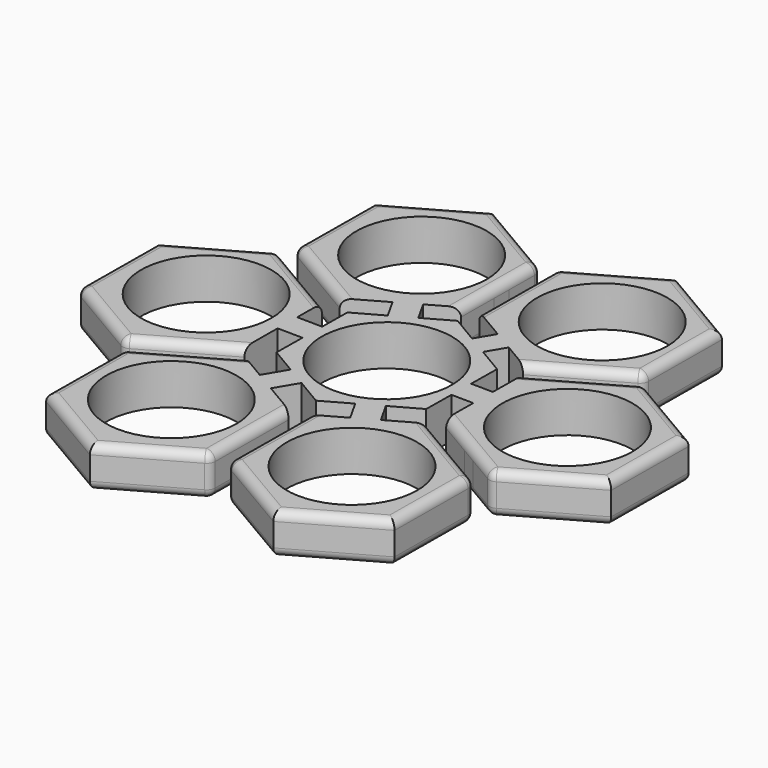
from build123d import *

# Parameters (mm, degrees)
F0_R          = 11.2
F1_DEPTH      = 7
F2_R          = 1.5
F3_R          = 1.5
F4_T1_DEPTH   = 19.3547728944
F4_T3_DEPTH   = 19.3547728944
F4_T5_DEPTH   = 19.3547728944
F4_T7_DEPTH   = 19.3547728944
F4_T9_DEPTH   = 19.3547728944
F4_T11_DEPTH  = 19.3547728944
F4_T13_DEPTH  = 19.3547728944
F4_T15_DEPTH  = 19.3547728944
F4_T17_DEPTH  = 19.3547728944
F4_T19_DEPTH  = 19.3547728944
F4_T21_DEPTH  = 19.3547728944
F4_T23_DEPTH  = 19.3547728944
F4_T25_DEPTH  = 4
F4_T27_DEPTH  = 7.6650635095
F4_T32_DEPTH  = 1.5
F4_T38_DEPTH  = 1.5
F4_T44_DEPTH  = 1.5
F4_T50_DEPTH  = 1.5
F4_T56_DEPTH  = 1.5
F4_T62_DEPTH  = 1.5
F4_T68_DEPTH  = 1.5
F4_T74_DEPTH  = 1.5
F4_T80_DEPTH  = 1.5
F4_T86_DEPTH  = 1.5
F4_T92_DEPTH  = 1.5
F4_T98_DEPTH  = 1.5
F4_T104_DEPTH = 1.5
F4_T110_DEPTH = 1.5
F4_T116_DEPTH = 1.5
F4_T122_DEPTH = 1.5
F4_T128_DEPTH = 1.5
F4_T134_DEPTH = 1.5
F4_T140_DEPTH = 1.5
F4_T146_DEPTH = 1.5
F4_T152_DEPTH = 1.5
F4_T158_DEPTH = 1.5
F4_T164_DEPTH = 1.5
F5_T1_DEPTH   = 14.7387474906
F5_T3_DEPTH   = 19.3547728944
F5_T5_DEPTH   = 4
F5_T10_DEPTH  = 1.5
F5_T16_DEPTH  = 1.5
F5_T20_ANGLE  = 60.0000000024


# Not quite as in the source:
# - a fillet or chamfer that OpenCascade refuses, or shapes differently, is made with other operations: its cross-section is extruded or revolved along the edge and cut away or added


with BuildPart() as f1:
    # F0 (on Top) → F1 (new body)
    with BuildSketch(Plane.XY):
        Polygon((-17.3645722709, -8.8701178063), (-17.3063848903, -1.7982007172), (-17.272166827, 2.3605585075), (-17.2290559521, 7.6001229905), (-25.7244198376, 12.5985677043), (-31.4249447291, 15.9526039637), (-45.7563498251, 7.8348441401), (-45.891866144, -8.6353966568), (-31.6959773669, -16.98787763), align=None)
        with Locations((-31.0137589486, 0)):
            Circle(F0_R, mode=Mode.SUBTRACT)
        Polygon((8.1018030655, -10.3313899594), (12.8824554247, -7.6483706617), (12.9474991031, -2.30788682), (12.9981476939, 1.8506722915), (13.064911003, 7.3323483301), (8.4724381667, 10.0589197287), (4.8963446285, 12.1820622508), (0.1824555782, 14.9807189918), (-4.4750609364, 12.3668065487), (-8.1018030655, 10.3313899594), (-12.8824554247, 7.6483706617), (-12.9474991031, 2.30788682), (-12.9981476939, -1.8506722915), (-13.064911003, -7.3323483301), (-8.4724381667, -10.0589197287), (-4.8963446285, -12.1820622508), (-0.1824555782, -14.9807189918), (4.4750609364, -12.3668065487), align=None)
        Circle(F0_R, mode=Mode.SUBTRACT)
        Polygon((-10.0334618511, 13.7732545552), (-6.4147616826, 15.8230004555), (-1.9451605955, 18.3547234715), (-1.8875629406, 25.354967087), (-1.8610559953, 28.5765405116), (-1.8096442766, 34.8249642683), (-16.0055330537, 43.1774452415), (-30.3369381496, 35.0596854179), (-30.4724544685, 18.589444621), (-16.2765656915, 10.2369636478), align=None)
        with Locations((-15.5068794743, 26.8587031163)):
            Circle(F0_R, mode=Mode.SUBTRACT)
        Polygon((6.7727997891, 15.3426504379), (10.3572818944, 13.2336371134), (15.0105443068, 10.4957820644), (21.1925256582, 13.9974512663), (23.9957435567, 15.5852822906), (29.3419494028, 18.613541888), (29.4774657217, 35.0837826849), (15.2815769446, 43.4362636581), (0.9501718486, 35.3185038344), (0.8146555298, 18.8482630376), align=None)
        with Locations((15.5068794743, 26.8587031163)):
            Circle(F0_R, mode=Mode.SUBTRACT)
        Polygon((16.7639962342, 1.8048066643), (16.729778171, -2.3539525605), (16.6823538526, -8.1177598236), (22.5808771528, -11.5882930469), (25.3575881061, -13.2220354473), (30.8782426297, -16.4702407968), (45.2096477256, -8.3524809732), (45.3451640445, 8.1177598236), (31.1492752675, 16.4702407968), (16.8178701715, 8.3524809732), align=None)
        with Locations((31.0137589486, 0)):
            Circle(F0_R, mode=Mode.SUBTRACT)
        Polygon((15.729863592, -10.754600481), (10.1220246336, -13.9310573245), (6.5033244651, -15.9808032248), (1.3984584961, -18.8723603046), (1.3451566516, -25.3505041951), (1.3186497063, -28.5720776198), (1.2629421772, -35.3426011014), (15.4588309543, -43.6950820746), (29.7902360502, -35.577322251), (29.9257523691, -19.1070814542), align=None)
        with Locations((15.5068794743, -26.8587031163)):
            Circle(F0_R, mode=Mode.SUBTRACT)
        Polygon((-1.3613576292, -19.3658998707), (-7.1420948508, -15.9646688233), (-10.726576956, -13.8556554989), (-15.5572464063, -11.0134188975), (-21.1033407868, -14.1549016649), (-23.9065586854, -15.7427326892), (-29.8886515022, -19.1311787212), (-30.0241678211, -35.601419518), (-15.828279044, -43.9539004912), (-1.4968739481, -35.8361406676), align=None)
        with Locations((-15.5068794743, -26.8587031163)):
            Circle(F0_R, mode=Mode.SUBTRACT)
        Polygon((-7.1420948508, -15.9646688233), (-4.8963446285, -12.1820622508), (-8.4724381667, -10.0589197287), (-10.726576956, -13.8556554989), align=None)
        Polygon((10.1220246336, -13.9310573245), (8.1018030655, -10.3313899594), (4.4750609364, -12.3668065487), (6.5033244651, -15.9808032248), align=None)
        Polygon((12.9981476939, 1.8506722915), (12.9474991031, -2.30788682), (16.729778171, -2.3539525605), (16.7639962342, 1.8048066643), align=None)
        Polygon((4.8963446285, 12.1820622508), (8.4724381667, 10.0589197287), (10.3572818944, 13.2336371134), (6.7727997891, 15.3426504379), align=None)
        Polygon((-8.1018030655, 10.3313899594), (-4.4750609364, 12.3668065487), (-6.4147616826, 15.8230004555), (-10.0334618511, 13.7732545552), align=None)
        Polygon((-17.3063848903, -1.7982007172), (-12.9981476939, -1.8506722915), (-12.9474991031, 2.30788682), (-17.272166827, 2.3605585075), align=None)
    extrude(amount=F1_DEPTH)

    # F2
    f2_edges = [f1.edges().sort_by_distance(p)[0] for p in [
        (22.624534, -39.636202, 7),
        (8.360887, -39.518842, 7),
        (-8.662576, -39.895021, 7),
        (-22.926223, -39.77766, 7),
        (-29.95641, -27.366299, 7),
        (-38.793922, -12.811637, 7),
        (-45.824108, -0.400276, 7),
        (-38.590647, 11.893724, 7),
        (-30.404696, 26.824565, 7),
        (-23.171236, 39.118565, 7),
        (-8.907589, 39.001205, 7),
        (8.115874, 39.377384, 7),
        (22.379521, 39.260023, 7),
        (38.24722, 12.294, 7),
        (29.409708, 26.848662, 7),
        (45.277406, -0.117361, 7),
        (38.043945, -12.411361, 7),
        (29.857994, -27.342202, 7),
    ]]
    fillet(f2_edges, radius=F2_R)

    # F3
    f3_edges = [f1.edges().sort_by_distance(p)[0] for p in [
        (-38.590647, 11.893724, 0),
        (-45.824108, -0.400276, 0),
        (-29.95641, -27.366299, 0),
        (-22.926223, -39.77766, 0),
        (-8.662576, -39.895021, 0),
        (8.360887, -39.518842, 0),
        (22.624534, -39.636202, 0),
        (29.857994, -27.342202, 0),
        (38.043945, -12.411361, 0),
        (45.277406, -0.117361, 0),
        (22.379521, 39.260023, 0),
        (38.24722, 12.294, 0),
        (29.409708, 26.848662, 0),
        (8.115874, 39.377384, 0),
        (-8.907589, 39.001205, 0),
        (-23.171236, 39.118565, 0),
        (-30.404696, 26.824565, 0),
    ]]
    fillet(f3_edges, radius=F3_R)

    # F4: fillet of radius 1.5 on 12 edges, made by hand

    # F4_s2 → F4_t1 (cut)
    with BuildSketch(Plane(origin=(-30.0146244367, 17.6598016131, 0), x_dir=(0, 0, 1), z_dir=(0.8618822549, -0.5071084487, 0))):
        with BuildLine():
            ThreePointArc((7, -2.0690733347), (6.5606601718, -1.0084131629), (5.5, -0.5690733347))
            Line((5.5, -0.5690733347), (7, -0.5690733347))
            Line((7, -0.5690733347), (7, -2.0690733347))
        make_face()
        with BuildLine():
            ThreePointArc((0, -2.0690733347), (0.4393398282, -1.0084131629), (1.5, -0.5690733347))
            Line((1.5, -0.5690733347), (0, -0.5690733347))
            Line((0, -0.5690733347), (0, -2.0690733347))
        make_face()
    extrude(amount=F4_T1_DEPTH, mode=Mode.SUBTRACT)

    # F4_s4 → F4_t3 (cut)
    with BuildSketch(Plane(origin=(0.1200260797, 14.5876042849, 0), x_dir=(0, 0, 1), z_dir=(0.0082276716, 0.9999661521, 0))):
        with BuildLine():
            ThreePointArc((7, -3.5961113925), (6.5606601718, -2.5354512207), (5.5, -2.0961113925))
            Line((5.5, -2.0961113925), (7, -2.0961113925))
            Line((7, -2.0961113925), (7, -3.5961113925))
        make_face()
        with BuildLine():
            ThreePointArc((0, -3.5961113925), (0.4393398282, -2.5354512207), (1.5, -2.0961113925))
            Line((1.5, -2.0961113925), (0, -2.0961113925))
            Line((0, -2.0961113925), (0, -3.5961113925))
        make_face()
    extrude(amount=F4_T3_DEPTH, mode=Mode.SUBTRACT)

    # F4_s6 → F4_t5 (cut)
    with BuildSketch(Plane(origin=(0.2835181629, 34.4579343098, 0), x_dir=(0, 0, 1), z_dir=(-0.0082276716, -0.9999661521, 0))):
        with BuildLine():
            ThreePointArc((7, -2.1595506375), (6.5606601718, -1.0988904657), (5.5, -0.6595506375))
            Line((5.5, -0.6595506375), (7, -0.6595506375))
            Line((7, -0.6595506375), (7, -2.1595506375))
        make_face()
        with BuildLine():
            ThreePointArc((0, -2.1595506375), (0.4393398282, -1.0988904657), (1.5, -0.6595506375))
            Line((1.5, -0.6595506375), (0, -0.6595506375))
            Line((0, -0.6595506375), (0, -2.1595506375))
        make_face()
    extrude(amount=F4_T5_DEPTH, mode=Mode.SUBTRACT)

    # F4_s8 → F4_t7 (cut)
    with BuildSketch(Plane(origin=(12.6024552107, 7.1384280818, 0), x_dir=(0, 0, 1), z_dir=(0.8701099265, 0.4928577035, 0))):
        with BuildLine():
            ThreePointArc((7, -3.2344217652), (6.5606601718, -2.1737615934), (5.5, -1.7344217652))
            Line((5.5, -1.7344217652), (7, -1.7344217652))
            Line((7, -1.7344217652), (7, -3.2344217652))
        make_face()
        with BuildLine():
            ThreePointArc((0, -3.2344217652), (0.4393398282, -2.1737615934), (1.5, -1.7344217652))
            Line((1.5, -1.7344217652), (0, -1.7344217652))
            Line((0, -1.7344217652), (0, -3.2344217652))
        make_face()
    extrude(amount=F4_T7_DEPTH, mode=Mode.SUBTRACT)

    # F4_s10 → F4_t9 (cut)
    with BuildSketch(Plane(origin=(29.8924118355, 16.9320047968, 0), x_dir=(0, 0, 1), z_dir=(-0.8701099265, -0.4928577035, 0))):
        with BuildLine():
            ThreePointArc((7, -2.5212402647), (6.5606601718, -1.460580093), (5.5, -1.0212402647))
            Line((5.5, -1.0212402647), (7, -1.0212402647))
            Line((7, -1.0212402647), (7, -2.5212402647))
        make_face()
        with BuildLine():
            ThreePointArc((0, -2.5212402647), (0.4393398282, -1.460580093), (1.5, -1.0212402647))
            Line((1.5, -1.0212402647), (0, -1.0212402647))
            Line((0, -1.0212402647), (0, -2.5212402647))
        make_face()
    extrude(amount=F4_T9_DEPTH, mode=Mode.SUBTRACT)

    # F4_s12 → F4_t11 (cut)
    with BuildSketch(Plane(origin=(12.7082895272, -7.4772173933, 0), x_dir=(0, 0, 1), z_dir=(0.8618822549, -0.5071084487, 0))):
        with BuildLine():
            ThreePointArc((7, -2.9632094408), (6.5606601718, -1.902549269), (5.5, -1.4632094408))
            Line((5.5, -1.4632094408), (7, -1.4632094408))
            Line((7, -1.4632094408), (7, -2.9632094408))
        make_face()
        with BuildLine():
            ThreePointArc((0, -2.9632094408), (0.4393398282, -1.902549269), (1.5, -1.4632094408))
            Line((1.5, -1.4632094408), (0, -1.4632094408))
            Line((0, -1.4632094408), (0, -2.9632094408))
        make_face()
    extrude(amount=F4_T11_DEPTH, mode=Mode.SUBTRACT)

    # F4_s14 → F4_t13 (cut)
    with BuildSketch(Plane(origin=(29.8347540687, -17.5539707032, 0), x_dir=(0, 0, 1), z_dir=(-0.8618822549, 0.5071084487, 0))):
        with BuildLine():
            ThreePointArc((7, -2.7924525892), (6.5606601718, -1.7317924174), (5.5, -1.2924525892))
            Line((5.5, -1.2924525892), (7, -1.2924525892))
            Line((7, -1.2924525892), (7, -2.7924525892))
        make_face()
        with BuildLine():
            ThreePointArc((0, -2.7924525892), (0.4393398282, -1.7317924174), (1.5, -1.2924525892))
            Line((1.5, -1.2924525892), (0, -1.2924525892))
            Line((0, -1.2924525892), (0, -2.7924525892))
        make_face()
    extrude(amount=F4_T13_DEPTH, mode=Mode.SUBTRACT)

    # F4_s16 → F4_t15 (cut)
    with BuildSketch(Plane(origin=(-0.1243218901, -15.1097040098, 0), x_dir=(0, 0, 1), z_dir=(-0.0082276716, -0.9999661521, 0))):
        with BuildLine():
            ThreePointArc((7, -3.0536867436), (6.5606601718, -1.9930265718), (5.5, -1.5536867436))
            Line((5.5, -1.5536867436), (7, -1.5536867436))
            Line((7, -1.5536867436), (7, -3.0536867436))
        make_face()
        with BuildLine():
            ThreePointArc((0, -3.0536867436), (0.4393398282, -1.9930265718), (1.5, -1.5536867436))
            Line((1.5, -1.5536867436), (0, -1.5536867436))
            Line((0, -1.5536867436), (0, -3.0536867436))
        make_face()
    extrude(amount=F4_T15_DEPTH, mode=Mode.SUBTRACT)

    # F4_s18 → F4_t17 (cut)
    with BuildSketch(Plane(origin=(-0.2878139734, -34.9800340348, 0), x_dir=(0, 0, 1), z_dir=(0.0082276716, 0.9999661521, 0))):
        with BuildLine():
            ThreePointArc((7, -2.7019752864), (6.5606601718, -1.6413151146), (5.5, -1.2019752864))
            Line((5.5, -1.2019752864), (7, -1.2019752864))
            Line((7, -1.2019752864), (7, -2.7019752864))
        make_face()
        with BuildLine():
            ThreePointArc((0, -2.7019752864), (0.4393398282, -1.6413151146), (1.5, -1.2019752864))
            Line((1.5, -1.2019752864), (0, -1.2019752864))
            Line((0, -1.2019752864), (0, -2.7019752864))
        make_face()
    extrude(amount=F4_T17_DEPTH, mode=Mode.SUBTRACT)

    # F4_s20 → F4_t19 (cut)
    with BuildSketch(Plane(origin=(-13.2383421815, -7.4986145164, 0), x_dir=(0, 0, 1), z_dir=(-0.8701099265, -0.4928577035, 0))):
        with BuildLine():
            ThreePointArc((5.5, -1.9153763708), (6.5606601718, -2.354716199), (7, -3.4153763708))
            Line((7, -3.4153763708), (7, -1.9153763708))
            Line((7, -1.9153763708), (5.5, -1.9153763708))
        make_face()
        with BuildLine():
            ThreePointArc((1.5, -1.9153763708), (0.4393398282, -2.354716199), (0, -3.4153763708))
            Line((0, -3.4153763708), (0, -1.9153763708))
            Line((0, -1.9153763708), (1.5, -1.9153763708))
        make_face()
    extrude(amount=F4_T19_DEPTH, mode=Mode.SUBTRACT)

    # F4_s22 → F4_t21 (cut)
    with BuildSketch(Plane(origin=(-30.5282988063, -17.2921912314, 0), x_dir=(0, 0, 1), z_dir=(0.8701099265, 0.4928577035, 0))):
        with BuildLine():
            ThreePointArc((7, -2.3402856591), (6.5606601718, -1.2796254874), (5.5, -0.8402856591))
            Line((5.5, -0.8402856591), (7, -0.8402856591))
            Line((7, -0.8402856591), (7, -2.3402856591))
        make_face()
    extrude(amount=F4_T21_DEPTH, mode=Mode.SUBTRACT)

    # F4_s24 → F4_t23 (cut)
    with BuildSketch(Plane(origin=(-12.8881598951, 7.5830483032, 0), x_dir=(0, 0, 1), z_dir=(-0.8618822549, 0.5071084487, 0))):
        with BuildLine():
            ThreePointArc((7, -3.6865886952), (6.5606601718, -2.6259285235), (5.5, -2.1865886952))
            Line((5.5, -2.1865886952), (7, -2.1865886952))
            Line((7, -2.1865886952), (7, -3.6865886952))
        make_face()
        with BuildLine():
            ThreePointArc((0, -3.6865886952), (0.4393398282, -2.6259285235), (1.5, -2.1865886952))
            Line((1.5, -2.1865886952), (0, -2.1865886952))
            Line((0, -2.1865886952), (0, -3.6865886952))
        make_face()
    extrude(amount=F4_T23_DEPTH, mode=Mode.SUBTRACT)

    # F4_s26 → F4_t25 (cut)
    with BuildSketch(Plane.XY.offset(1.5)):
        with BuildLine():
            ThreePointArc((-30.6785328013, 15.5134351647), (-31.426853967, 15.7205610106), (-32.1784820295, 15.5257766721))
            Line((-32.1784820295, 15.5257766721), (-31.4249447291, 15.9526039637))
            Line((-31.4249447291, 15.9526039637), (-30.6785328013, 15.5134351647))
        make_face()
        with BuildLine():
            ThreePointArc((-29.1351142018, -18.7043514295), (-29.688651029, -19.2488536462), (-29.8957768748, -19.9971748118))
            Line((-29.8957768748, -19.9971748118), (-29.8886515022, -19.1311787212))
            Line((-29.8886515022, -19.1311787212), (-29.1351142018, -18.7043514295))
        make_face()
        with BuildLine():
            ThreePointArc((-1.4897485755, -34.9701445769), (-1.6968744214, -35.7184657425), (-2.2504112485, -36.2629679592))
            Line((-2.2504112485, -36.2629679592), (-1.4968739481, -35.8361406676))
            Line((-1.4968739481, -35.8361406676), (-1.4897485755, -34.9701445769))
        make_face()
        with BuildLine():
            ThreePointArc((1.2700675498, -34.4766050108), (1.4648518883, -35.2282330733), (2.009354105, -35.7817699005))
            Line((2.009354105, -35.7817699005), (1.2629421772, -35.3426011014))
            Line((1.2629421772, -35.3426011014), (1.2700675498, -34.4766050108))
        make_face()
        with BuildLine():
            ThreePointArc((29.1793404413, -18.6679126551), (29.723842658, -19.2214494823), (29.9186269965, -19.9730775448))
            Line((29.9186269965, -19.9730775448), (29.9257523691, -19.1070814542))
            Line((29.9257523691, -19.1070814542), (29.1793404413, -18.6679126551))
        make_face()
        with BuildLine():
            ThreePointArc((30.1318307019, -16.0310719978), (30.8801518675, -16.2381978437), (31.6317799301, -16.0434135052))
            Line((31.6317799301, -16.0434135052), (30.8782426297, -16.4702407968))
            Line((30.8782426297, -16.4702407968), (30.1318307019, -16.0310719978))
        make_face()
        with BuildLine():
            ThreePointArc((30.3957379671, 16.0434135052), (31.1473660296, 16.2381978437), (31.8956871953, 16.0310719978))
            Line((31.8956871953, 16.0310719978), (31.1492752675, 16.4702407968))
            Line((31.1492752675, 16.4702407968), (30.3957379671, 16.0434135052))
        make_face()
        with BuildLine():
            ThreePointArc((28.5884121024, 18.1867145964), (29.1419489295, 18.7312168131), (29.3490747754, 19.4795379787))
            Line((29.3490747754, 19.4795379787), (29.3419494028, 18.613541888))
            Line((29.3419494028, 18.613541888), (28.5884121024, 18.1867145964))
        make_face()
        with BuildLine():
            ThreePointArc((0.9430464761, 34.4525077438), (1.1501723219, 35.2008289094), (1.703709149, 35.7453311261))
            Line((1.703709149, 35.7453311261), (0.9501718486, 35.3185038344))
            Line((0.9501718486, 35.3185038344), (0.9430464761, 34.4525077438))
        make_face()
        with BuildLine():
            ThreePointArc((-1.8167696492, 33.9589681776), (-2.0115539877, 34.7105962402), (-2.5560562044, 35.2641330673))
            Line((-2.5560562044, 35.2641330673), (-1.8096442766, 34.8249642683))
            Line((-1.8096442766, 34.8249642683), (-1.8167696492, 33.9589681776))
        make_face()
        with BuildLine():
            ThreePointArc((-29.7260425407, 18.150275822), (-30.2705447574, 18.7038126491), (-30.4653290959, 19.4554407117))
            Line((-30.4653290959, 19.4554407117), (-30.4724544685, 18.589444621))
            Line((-30.4724544685, 18.589444621), (-29.7260425407, 18.150275822))
        make_face()
    extrude(amount=F4_T25_DEPTH, mode=Mode.SUBTRACT)

    # F4_s28 → F4_t27 (cut)
    with BuildSketch(Plane.XY.offset(-2.1650635095)):
        with BuildLine():
            ThreePointArc((-30.9424400665, -16.5610503383), (-31.6940681291, -16.7558346768), (-32.4423892947, -16.5487088309))
            Line((-32.4423892947, -16.5487088309), (-31.6959773669, -16.98787763))
            Line((-31.6959773669, -16.98787763), (-30.9424400665, -16.5610503383))
        make_face()
    extrude(amount=F4_T27_DEPTH, mode=Mode.SUBTRACT)


with BuildPart() as f4_tool30:
    # F4_s31 → F4_t32 (new body)
    with BuildSketch(Plane.XY.offset(5.5)):
        Polygon((-31.4391954743, 14.2206117824), (-32.1784820295, 15.5257766721), (-31.4249447291, 15.9526039637), (-30.6785328013, 15.5134351647), align=None)
    extrude(amount=F4_T32_DEPTH)

    # F4_s33 → F4_t34 (revolve, cut)
    with BuildSketch(Plane(origin=(-31.4391954743, 14.2206117824, 5.5), x_dir=(-0.0082276716, -0.9999661521, 0), z_dir=(-0.9999661521, 0.0082276716, 0))):
        with BuildLine():
            ThreePointArc((0, -1.5), (1.5, 0), (0, 1.5))
            Line((0, 1.5), (0, -1.5))
        make_face()
    revolve(axis=Axis((-31.4391954743, 14.2206117824, 5.5), (0, 0, 1)), mode=Mode.SUBTRACT)


with BuildPart() as f1_1:
    add(f1.part)

    # F4_t29: cut F4_tool30
    add(f4_tool30.part, mode=Mode.SUBTRACT)


with BuildPart() as f4_tool36:
    # F4_s37 → F4_t38 (new body)
    with BuildSketch(Plane.XY.offset(1.5)):
        Polygon((-31.4391954743, 14.2206117824), (-30.6785328013, 15.5134351647), (-31.4249447291, 15.9526039637), (-32.1784820295, 15.5257766721), align=None)
    extrude(amount=-F4_T38_DEPTH)

    # F4_s39 → F4_t40 (revolve, cut)
    with BuildSketch(Plane(origin=(-31.4391954743, 14.2206117824, 1.5), x_dir=(-0.0082276716, -0.9999661521, 0), z_dir=(0.9999661521, -0.0082276716, 0))):
        with BuildLine():
            ThreePointArc((0, -1.5), (1.5, 0), (0, 1.5))
            Line((0, 1.5), (0, -1.5))
        make_face()
    revolve(axis=Axis((-31.4391954743, 14.2206117824, 1.5), (0, 0, -1)), mode=Mode.SUBTRACT)


with BuildPart() as f1_2:
    add(f1_1.part)

    # F4_t35: cut F4_tool36
    add(f4_tool36.part, mode=Mode.SUBTRACT)


with BuildPart() as f4_tool42:
    # F4_s43 → F4_t44 (new body)
    with BuildSketch(Plane.XY.offset(5.5)):
        Polygon((-31.6817266217, -15.2558854486), (-32.4423892947, -16.5487088309), (-31.6959773669, -16.98787763), (-30.9424400665, -16.5610503383), align=None)
    extrude(amount=F4_T44_DEPTH)

    # F4_s45 → F4_t46 (revolve, cut)
    with BuildSketch(Plane(origin=(-31.6817266217, -15.2558854486, 5.5), x_dir=(0.0082276716, 0.9999661521, 0), z_dir=(0.9999661521, -0.0082276716, 0))):
        with BuildLine():
            ThreePointArc((0, -1.5), (1.5, 0), (0, 1.5))
            Line((0, 1.5), (0, -1.5))
        make_face()
    revolve(axis=Axis((-31.6817266217, -15.2558854486, 5.5), (0, 0, 1)), mode=Mode.SUBTRACT)


with BuildPart() as f1_3:
    add(f1_2.part)

    # F4_t41: cut F4_tool42
    add(f4_tool42.part, mode=Mode.SUBTRACT)


with BuildPart() as f4_tool48:
    # F4_s49 → F4_t50 (new body)
    with BuildSketch(Plane.XY.offset(5.5)):
        Polygon((-28.3958276466, -20.0095163192), (-29.1351142018, -18.7043514295), (-29.8886515022, -19.1311787212), (-29.8957768748, -19.9971748118), align=None)
    extrude(amount=F4_T50_DEPTH)

    # F4_s51 → F4_t52 (revolve, cut)
    with BuildSketch(Plane(origin=(-28.3958276466, -20.0095163192, 5.5), x_dir=(0.8618822549, -0.5071084487, 0), z_dir=(-0.5071084487, -0.8618822549, 0))):
        with BuildLine():
            ThreePointArc((0, -1.5), (1.5, 0), (0, 1.5))
            Line((0, 1.5), (0, -1.5))
        make_face()
    revolve(axis=Axis((-28.3958276466, -20.0095163192, 5.5), (0, 0, 1)), mode=Mode.SUBTRACT)


with BuildPart() as f1_4:
    add(f1_3.part)

    # F4_t47: cut F4_tool48
    add(f4_tool48.part, mode=Mode.SUBTRACT)


with BuildPart() as f4_tool54:
    # F4_s55 → F4_t56 (new body)
    with BuildSketch(Plane.XY.offset(1.5)):
        Polygon((-28.3958276466, -20.0095163192), (-29.1351142018, -18.7043514295), (-29.8886515022, -19.1311787212), (-29.8957768748, -19.9971748118), align=None)
    extrude(amount=-F4_T56_DEPTH)

    # F4_s57 → F4_t58 (revolve, cut)
    with BuildSketch(Plane(origin=(-28.3958276466, -20.0095163192, 1.5), x_dir=(0.8618822549, -0.5071084487, 0), z_dir=(0.5071084487, 0.8618822549, 0))):
        with BuildLine():
            ThreePointArc((0, -1.5), (1.5, 0), (0, 1.5))
            Line((0, 1.5), (0, -1.5))
        make_face()
    revolve(axis=Axis((-28.3958276466, -20.0095163192, 1.5), (0, 0, -1)), mode=Mode.SUBTRACT)


with BuildPart() as f1_5:
    add(f1_4.part)

    # F4_t53: cut F4_tool54
    add(f4_tool54.part, mode=Mode.SUBTRACT)


with BuildPart() as f4_tool60:
    # F4_s61 → F4_t62 (new body)
    with BuildSketch(Plane.XY.offset(5.5)):
        Polygon((-2.9896978037, -34.9578030695), (-1.4897485755, -34.9701445769), (-1.4968739481, -35.8361406676), (-2.2504112485, -36.2629679592), align=None)
    extrude(amount=F4_T62_DEPTH)

    # F4_s63 → F4_t64 (revolve, cut)
    with BuildSketch(Plane(origin=(-2.9896978037, -34.9578030695, 5.5), x_dir=(-0.8618822549, 0.5071084487, 0), z_dir=(0.5071084487, 0.8618822549, 0))):
        with BuildLine():
            ThreePointArc((0, -1.5), (1.5, 0), (0, 1.5))
            Line((0, 1.5), (0, -1.5))
        make_face()
    revolve(axis=Axis((-2.9896978037, -34.9578030695, 5.5), (0, 0, 1)), mode=Mode.SUBTRACT)


with BuildPart() as f1_6:
    add(f1_5.part)

    # F4_t59: cut F4_tool60
    add(f4_tool60.part, mode=Mode.SUBTRACT)


with BuildPart() as f4_tool66:
    # F4_s67 → F4_t68 (new body)
    with BuildSketch(Plane.XY.offset(1.5)):
        Polygon((-2.9896978037, -34.9578030695), (-1.4897485755, -34.9701445769), (-1.4968739481, -35.8361406676), (-2.2504112485, -36.2629679592), align=None)
    extrude(amount=-F4_T68_DEPTH)

    # F4_s69 → F4_t70 (revolve, cut)
    with BuildSketch(Plane(origin=(-2.9896978037, -34.9578030695, 1.5), x_dir=(-0.8618822549, 0.5071084487, 0), z_dir=(-0.5071084487, -0.8618822549, 0))):
        with BuildLine():
            ThreePointArc((0, -1.5), (1.5, 0), (0, 1.5))
            Line((0, 1.5), (0, -1.5))
        make_face()
    revolve(axis=Axis((-2.9896978037, -34.9578030695, 1.5), (0, 0, -1)), mode=Mode.SUBTRACT)


with BuildPart() as f1_7:
    add(f1_6.part)

    # F4_t65: cut F4_tool66
    add(f4_tool66.part, mode=Mode.SUBTRACT)


with BuildPart() as f4_tool72:
    # F4_s73 → F4_t74 (new body)
    with BuildSketch(Plane.XY.offset(5.5)):
        Polygon((2.770016778, -34.4889465181), (2.009354105, -35.7817699005), (1.2629421772, -35.3426011014), (1.2700675498, -34.4766050108), align=None)
    extrude(amount=F4_T74_DEPTH)

    # F4_s75 → F4_t76 (revolve, cut)
    with BuildSketch(Plane(origin=(2.770016778, -34.4889465181, 5.5), x_dir=(0.8701099265, 0.4928577035, 0), z_dir=(0.4928577035, -0.8701099265, 0))):
        with BuildLine():
            ThreePointArc((0, -1.5), (1.5, 0), (0, 1.5))
            Line((0, 1.5), (0, -1.5))
        make_face()
    revolve(axis=Axis((2.770016778, -34.4889465181, 5.5), (0, 0, 1)), mode=Mode.SUBTRACT)


with BuildPart() as f1_8:
    add(f1_7.part)

    # F4_t71: cut F4_tool72
    add(f4_tool72.part, mode=Mode.SUBTRACT)


with BuildPart() as f4_tool78:
    # F4_s79 → F4_t80 (new body)
    with BuildSketch(Plane.XY.offset(1.5)):
        Polygon((2.770016778, -34.4889465181), (2.009354105, -35.7817699005), (1.2629421772, -35.3426011014), (1.2700675498, -34.4766050108), align=None)
    extrude(amount=-F4_T80_DEPTH)

    # F4_s81 → F4_t82 (revolve, cut)
    with BuildSketch(Plane(origin=(2.770016778, -34.4889465181, 1.5), x_dir=(0.8701099265, 0.4928577035, 0), z_dir=(-0.4928577035, 0.8701099265, 0))):
        with BuildLine():
            ThreePointArc((0, -1.5), (1.5, 0), (0, 1.5))
            Line((0, 1.5), (0, -1.5))
        make_face()
    revolve(axis=Axis((2.770016778, -34.4889465181, 1.5), (0, 0, -1)), mode=Mode.SUBTRACT)


with BuildPart() as f1_9:
    add(f1_8.part)

    # F4_t77: cut F4_tool78
    add(f4_tool78.part, mode=Mode.SUBTRACT)


with BuildPart() as f4_tool84:
    # F4_s85 → F4_t86 (new body)
    with BuildSketch(Plane.XY.offset(5.5)):
        Polygon((28.4186777683, -19.9607360375), (29.1793404413, -18.6679126551), (29.9257523691, -19.1070814542), (29.9186269965, -19.9730775448), align=None)
    extrude(amount=F4_T86_DEPTH)

    # F4_s87 → F4_t88 (revolve, cut)
    with BuildSketch(Plane(origin=(28.4186777683, -19.9607360375, 5.5), x_dir=(-0.8701099265, -0.4928577035, 0), z_dir=(-0.4928577035, 0.8701099265, 0))):
        with BuildLine():
            ThreePointArc((0, -1.5), (1.5, 0), (0, 1.5))
            Line((0, 1.5), (0, -1.5))
        make_face()
    revolve(axis=Axis((28.4186777683, -19.9607360375, 5.5), (0, 0, 1)), mode=Mode.SUBTRACT)


with BuildPart() as f1_10:
    add(f1_9.part)

    # F4_t83: cut F4_tool84
    add(f4_tool84.part, mode=Mode.SUBTRACT)


with BuildPart() as f4_tool90:
    # F4_s91 → F4_t92 (new body)
    with BuildSketch(Plane.XY.offset(1.5)):
        Polygon((28.4186777683, -19.9607360375), (29.9186269965, -19.9730775448), (29.9257523691, -19.1070814542), (29.1793404413, -18.6679126551), align=None)
    extrude(amount=-F4_T92_DEPTH)

    # F4_s93 → F4_t94 (revolve, cut)
    with BuildSketch(Plane(origin=(28.4186777683, -19.9607360375, 1.5), x_dir=(-0.8701099265, -0.4928577035, 0), z_dir=(0.4928577035, -0.8701099265, 0))):
        with BuildLine():
            ThreePointArc((0, -1.5), (1.5, 0), (0, 1.5))
            Line((0, 1.5), (0, -1.5))
        make_face()
    revolve(axis=Axis((28.4186777683, -19.9607360375, 1.5), (0, 0, -1)), mode=Mode.SUBTRACT)


with BuildPart() as f1_11:
    add(f1_10.part)

    # F4_t89: cut F4_tool90
    add(f4_tool90.part, mode=Mode.SUBTRACT)


with BuildPart() as f4_tool96:
    # F4_s97 → F4_t98 (new body)
    with BuildSketch(Plane.XY.offset(5.5)):
        Polygon((30.8924933749, -14.7382486155), (31.6317799301, -16.0434135052), (30.8782426297, -16.4702407968), (30.1318307019, -16.0310719978), align=None)
    extrude(amount=F4_T98_DEPTH)

    # F4_s99 → F4_t100 (revolve, cut)
    with BuildSketch(Plane(origin=(30.8924933749, -14.7382486155, 5.5), x_dir=(0.0082276716, 0.9999661521, 0), z_dir=(0.9999661521, -0.0082276716, 0))):
        with BuildLine():
            ThreePointArc((0, -1.5), (1.5, 0), (0, 1.5))
            Line((0, 1.5), (0, -1.5))
        make_face()
    revolve(axis=Axis((30.8924933749, -14.7382486155, 5.5), (0, 0, 1)), mode=Mode.SUBTRACT)


with BuildPart() as f1_12:
    add(f1_11.part)

    # F4_t95: cut F4_tool96
    add(f4_tool96.part, mode=Mode.SUBTRACT)


with BuildPart() as f4_tool102:
    # F4_s103 → F4_t104 (new body)
    with BuildSketch(Plane.XY.offset(1.5)):
        Polygon((30.8924933749, -14.7382486155), (31.6317799301, -16.0434135052), (30.8782426297, -16.4702407968), (30.1318307019, -16.0310719978), align=None)
    extrude(amount=-F4_T104_DEPTH)

    # F4_s105 → F4_t106 (revolve, cut)
    with BuildSketch(Plane(origin=(30.8924933749, -14.7382486155, 1.5), x_dir=(0.0082276716, 0.9999661521, 0), z_dir=(-0.9999661521, 0.0082276716, 0))):
        with BuildLine():
            ThreePointArc((0, -1.5), (1.5, 0), (0, 1.5))
            Line((0, 1.5), (0, -1.5))
        make_face()
    revolve(axis=Axis((30.8924933749, -14.7382486155, 1.5), (0, 0, -1)), mode=Mode.SUBTRACT)


with BuildPart() as f1_13:
    add(f1_12.part)

    # F4_t101: cut F4_tool102
    add(f4_tool102.part, mode=Mode.SUBTRACT)


with BuildPart() as f4_tool108:
    # F4_s109 → F4_t110 (new body)
    with BuildSketch(Plane.XY.offset(5.5)):
        Polygon((31.1350245223, 14.7382486155), (30.3957379671, 16.0434135052), (31.1492752675, 16.4702407968), (31.8956871953, 16.0310719978), align=None)
    extrude(amount=F4_T110_DEPTH)

    # F4_s111 → F4_t112 (revolve, cut)
    with BuildSketch(Plane(origin=(31.1350245223, 14.7382486155, 5.5), x_dir=(-0.0082276716, -0.9999661521, 0), z_dir=(-0.9999661521, 0.0082276716, 0))):
        with BuildLine():
            ThreePointArc((0, -1.5), (1.5, 0), (0, 1.5))
            Line((0, 1.5), (0, -1.5))
        make_face()
    revolve(axis=Axis((31.1350245223, 14.7382486155, 5.5), (0, 0, 1)), mode=Mode.SUBTRACT)


with BuildPart() as f1_14:
    add(f1_13.part)

    # F4_t107: cut F4_tool108
    add(f4_tool108.part, mode=Mode.SUBTRACT)


with BuildPart() as f4_tool114:
    # F4_s115 → F4_t116 (new body)
    with BuildSketch(Plane.XY.offset(1.5)):
        Polygon((31.1350245223, 14.7382486155), (30.3957379671, 16.0434135052), (31.1492752675, 16.4702407968), (31.8956871953, 16.0310719978), align=None)
    extrude(amount=-F4_T116_DEPTH)

    # F4_s117 → F4_t118 (revolve, cut)
    with BuildSketch(Plane(origin=(31.1350245223, 14.7382486155, 1.5), x_dir=(-0.0082276716, -0.9999661521, 0), z_dir=(0.9999661521, -0.0082276716, 0))):
        with BuildLine():
            ThreePointArc((0, -1.5), (1.5, 0), (0, 1.5))
            Line((0, 1.5), (0, -1.5))
        make_face()
    revolve(axis=Axis((31.1350245223, 14.7382486155, 1.5), (0, 0, -1)), mode=Mode.SUBTRACT)


with BuildPart() as f1_15:
    add(f1_14.part)

    # F4_t113: cut F4_tool114
    add(f4_tool114.part, mode=Mode.SUBTRACT)


with BuildPart() as f4_tool120:
    # F4_s121 → F4_t122 (new body)
    with BuildSketch(Plane.XY.offset(5.5)):
        Polygon((27.8491255472, 19.4918794861), (29.3490747754, 19.4795379787), (29.3419494028, 18.613541888), (28.5884121024, 18.1867145964), align=None)
    extrude(amount=F4_T122_DEPTH)

    # F4_s123 → F4_t124 (revolve, cut)
    with BuildSketch(Plane(origin=(27.8491255472, 19.4918794861, 5.5), x_dir=(-0.8618822549, 0.5071084487, 0), z_dir=(0.5071084487, 0.8618822549, 0))):
        with BuildLine():
            ThreePointArc((0, -1.5), (1.5, 0), (0, 1.5))
            Line((0, 1.5), (0, -1.5))
        make_face()
    revolve(axis=Axis((27.8491255472, 19.4918794861, 5.5), (0, 0, 1)), mode=Mode.SUBTRACT)


with BuildPart() as f1_16:
    add(f1_15.part)

    # F4_t119: cut F4_tool120
    add(f4_tool120.part, mode=Mode.SUBTRACT)


with BuildPart() as f4_tool126:
    # F4_s127 → F4_t128 (new body)
    with BuildSketch(Plane.XY.offset(1.5)):
        Polygon((27.8491255472, 19.4918794861), (29.3490747754, 19.4795379787), (29.3419494028, 18.613541888), (28.5884121024, 18.1867145964), align=None)
    extrude(amount=-F4_T128_DEPTH)

    # F4_s129 → F4_t130 (revolve, cut)
    with BuildSketch(Plane(origin=(27.8491255472, 19.4918794861, 1.5), x_dir=(-0.8618822549, 0.5071084487, 0), z_dir=(-0.5071084487, -0.8618822549, 0))):
        with BuildLine():
            ThreePointArc((0, -1.5), (1.5, 0), (0, 1.5))
            Line((0, 1.5), (0, -1.5))
        make_face()
    revolve(axis=Axis((27.8491255472, 19.4918794861, 1.5), (0, 0, -1)), mode=Mode.SUBTRACT)


with BuildPart() as f1_17:
    add(f1_16.part)

    # F4_t125: cut F4_tool126
    add(f4_tool126.part, mode=Mode.SUBTRACT)


with BuildPart() as f4_tool132:
    # F4_s133 → F4_t134 (new body)
    with BuildSketch(Plane.XY.offset(5.5)):
        Polygon((2.4429957043, 34.4401662364), (0.9430464761, 34.4525077438), (0.9501718486, 35.3185038344), (1.703709149, 35.7453311261), align=None)
    extrude(amount=F4_T134_DEPTH)

    # F4_s135 → F4_t136 (revolve, cut)
    with BuildSketch(Plane(origin=(2.4429957043, 34.4401662364, 5.5), x_dir=(0.8618822549, -0.5071084487, 0), z_dir=(-0.5071084487, -0.8618822549, 0))):
        with BuildLine():
            ThreePointArc((0, -1.5), (1.5, 0), (0, 1.5))
            Line((0, 1.5), (0, -1.5))
        make_face()
    revolve(axis=Axis((2.4429957043, 34.4401662364, 5.5), (0, 0, 1)), mode=Mode.SUBTRACT)


with BuildPart() as f1_18:
    add(f1_17.part)

    # F4_t131: cut F4_tool132
    add(f4_tool132.part, mode=Mode.SUBTRACT)


with BuildPart() as f4_tool138:
    # F4_s139 → F4_t140 (new body)
    with BuildSketch(Plane.XY.offset(1.5)):
        Polygon((2.4429957043, 34.4401662364), (0.9430464761, 34.4525077438), (0.9501718486, 35.3185038344), (1.703709149, 35.7453311261), align=None)
    extrude(amount=-F4_T140_DEPTH)

    # F4_s141 → F4_t142 (revolve, cut)
    with BuildSketch(Plane(origin=(2.4429957043, 34.4401662364, 1.5), x_dir=(0.8618822549, -0.5071084487, 0), z_dir=(0.5071084487, 0.8618822549, 0))):
        with BuildLine():
            ThreePointArc((0, -1.5), (1.5, 0), (0, 1.5))
            Line((0, 1.5), (0, -1.5))
        make_face()
    revolve(axis=Axis((2.4429957043, 34.4401662364, 1.5), (0, 0, -1)), mode=Mode.SUBTRACT)


with BuildPart() as f1_19:
    add(f1_18.part)

    # F4_t137: cut F4_tool138
    add(f4_tool138.part, mode=Mode.SUBTRACT)


with BuildPart() as f4_tool144:
    # F4_s145 → F4_t146 (new body)
    with BuildSketch(Plane.XY.offset(5.5)):
        Polygon((-3.3167188774, 33.971309685), (-2.5560562044, 35.2641330673), (-1.8096442766, 34.8249642683), (-1.8167696492, 33.9589681776), align=None)
    extrude(amount=F4_T146_DEPTH)

    # F4_s147 → F4_t148 (revolve, cut)
    with BuildSketch(Plane(origin=(-3.3167188774, 33.971309685, 5.5), x_dir=(-0.8701099265, -0.4928577035, 0), z_dir=(-0.4928577035, 0.8701099265, 0))):
        with BuildLine():
            ThreePointArc((0, -1.5), (1.5, 0), (0, 1.5))
            Line((0, 1.5), (0, -1.5))
        make_face()
    revolve(axis=Axis((-3.3167188774, 33.971309685, 5.5), (0, 0, 1)), mode=Mode.SUBTRACT)


with BuildPart() as f1_20:
    add(f1_19.part)

    # F4_t143: cut F4_tool144
    add(f4_tool144.part, mode=Mode.SUBTRACT)


with BuildPart() as f4_tool150:
    # F4_s151 → F4_t152 (new body)
    with BuildSketch(Plane.XY.offset(1.5)):
        Polygon((-3.3167188774, 33.971309685), (-2.5560562044, 35.2641330673), (-1.8096442766, 34.8249642683), (-1.8167696492, 33.9589681776), align=None)
    extrude(amount=-F4_T152_DEPTH)

    # F4_s153 → F4_t154 (revolve, cut)
    with BuildSketch(Plane(origin=(-3.3167188774, 33.971309685, 1.5), x_dir=(-0.8701099265, -0.4928577035, 0), z_dir=(0.4928577035, -0.8701099265, 0))):
        with BuildLine():
            ThreePointArc((0, -1.5), (1.5, 0), (0, 1.5))
            Line((0, 1.5), (0, -1.5))
        make_face()
    revolve(axis=Axis((-3.3167188774, 33.971309685, 1.5), (0, 0, -1)), mode=Mode.SUBTRACT)


with BuildPart() as f1_21:
    add(f1_20.part)

    # F4_t149: cut F4_tool150
    add(f4_tool150.part, mode=Mode.SUBTRACT)


with BuildPart() as f4_tool156:
    # F4_s157 → F4_t158 (new body)
    with BuildSketch(Plane.XY.offset(5.5)):
        Polygon((-28.9653798677, 19.4430992044), (-30.4653290959, 19.4554407117), (-30.4724544685, 18.589444621), (-29.7260425407, 18.150275822), align=None)
    extrude(amount=F4_T158_DEPTH)

    # F4_s159 → F4_t160 (revolve, cut)
    with BuildSketch(Plane(origin=(-28.9653798677, 19.4430992044, 5.5), x_dir=(0.8701099265, 0.4928577035, 0), z_dir=(0.4928577035, -0.8701099265, 0))):
        with BuildLine():
            ThreePointArc((0, -1.5), (1.5, 0), (0, 1.5))
            Line((0, 1.5), (0, -1.5))
        make_face()
    revolve(axis=Axis((-28.9653798677, 19.4430992044, 5.5), (0, 0, 1)), mode=Mode.SUBTRACT)


with BuildPart() as f1_22:
    add(f1_21.part)

    # F4_t155: cut F4_tool156
    add(f4_tool156.part, mode=Mode.SUBTRACT)


with BuildPart() as f4_tool162:
    # F4_s163 → F4_t164 (new body)
    with BuildSketch(Plane.XY.offset(1.5)):
        Polygon((-28.9653798677, 19.4430992044), (-30.4653290959, 19.4554407117), (-30.4724544685, 18.589444621), (-29.7260425407, 18.150275822), align=None)
    extrude(amount=-F4_T164_DEPTH)

    # F4_s165 → F4_t166 (revolve, cut)
    with BuildSketch(Plane(origin=(-28.9653798677, 19.4430992044, 1.5), x_dir=(0.8701099265, 0.4928577035, 0), z_dir=(-0.4928577035, 0.8701099265, 0))):
        with BuildLine():
            ThreePointArc((0, -1.5), (1.5, 0), (0, 1.5))
            Line((0, 1.5), (0, -1.5))
        make_face()
    revolve(axis=Axis((-28.9653798677, 19.4430992044, 1.5), (0, 0, -1)), mode=Mode.SUBTRACT)


with BuildPart() as f1_23:
    add(f1_22.part)

    # F4_t161: cut F4_tool162
    add(f4_tool162.part, mode=Mode.SUBTRACT)

    # F5: fillet of radius 1.5 on 4 edges, made by hand

    # F5_s2 → F5_t1 (cut)
    with BuildSketch(Plane(origin=(-29.5696952002, 17.3980171599, 0), x_dir=(0, 0, 1), z_dir=(0.8618822549, -0.5071084487, 0))):
        with BuildLine():
            ThreePointArc((0, 29.2148481889), (0.4393398282, 30.2755083606), (1.5, 30.7148481889))
            Line((1.5, 30.7148481889), (0, 30.7148481889))
            Line((0, 30.7148481889), (0, 29.2148481889))
        make_face()
    extrude(amount=F5_T1_DEPTH, mode=Mode.SUBTRACT)

    # F5_s4 → F5_t3 (cut)
    with BuildSketch(Plane(origin=(-30.5282988063, -17.2921912314, 0), x_dir=(0, 0, 1), z_dir=(0.8701099265, 0.4928577035, 0))):
        with BuildLine():
            ThreePointArc((0, -2.3402856591), (0.4393398282, -1.2796254874), (1.5, -0.8402856591))
            Line((1.5, -0.8402856591), (0, -0.8402856591))
            Line((0, -0.8402856591), (0, -2.3402856591))
        make_face()
    extrude(amount=F5_T3_DEPTH, mode=Mode.SUBTRACT)

    # F5_s6 → F5_t5 (cut)
    with BuildSketch(Plane.XY.offset(1.5)):
        with BuildLine():
            ThreePointArc((-45.1454542162, -9.0745654558), (-45.6899564329, -8.5210286287), (-45.8847407714, -7.7694005661))
            Line((-45.8847407714, -7.7694005661), (-45.891866144, -8.6353966568))
            Line((-45.891866144, -8.6353966568), (-45.1454542162, -9.0745654558))
        make_face()
    extrude(amount=F5_T5_DEPTH, mode=Mode.SUBTRACT)


with BuildPart() as f5_tool8:
    # F5_s9 → F5_t10 (new body)
    with BuildSketch(Plane.XY.offset(5.5)):
        Polygon((-44.3847915432, -7.7817420734), (-45.1454542162, -9.0745654558), (-45.891866144, -8.6353966568), (-45.8847407714, -7.7694005661), align=None)
    extrude(amount=F5_T10_DEPTH)

    # F5_s11 → F5_t12 (revolve, cut)
    with BuildSketch(Plane(origin=(-44.3847915432, -7.7817420734, 5.5), x_dir=(0.8701099265, 0.4928577035, 0), z_dir=(0.4928577035, -0.8701099265, 0))):
        with BuildLine():
            ThreePointArc((0, -1.5), (1.5, 0), (0, 1.5))
            Line((0, 1.5), (0, -1.5))
        make_face()
    revolve(axis=Axis((-44.3847915432, -7.7817420734, 5.5), (0, 0, 1)), mode=Mode.SUBTRACT)


with BuildPart() as f1_24:
    add(f1_23.part)

    # F5_t7: cut F5_tool8
    add(f5_tool8.part, mode=Mode.SUBTRACT)


with BuildPart() as f5_tool14:
    # F5_s15 → F5_t16 (new body)
    with BuildSketch(Plane.XY.offset(1.5)):
        Polygon((-44.3847915432, -7.7817420734), (-45.1454542162, -9.0745654558), (-45.891866144, -8.6353966568), (-45.8847407714, -7.7694005661), align=None)
    extrude(amount=-F5_T16_DEPTH)

    # F5_s17 → F5_t18 (revolve, cut)
    with BuildSketch(Plane(origin=(-44.3847915432, -7.7817420734, 1.5), x_dir=(0.8701099265, 0.4928577035, 0), z_dir=(-0.4928577035, 0.8701099265, 0))):
        with BuildLine():
            ThreePointArc((0, -1.5), (1.5, 0), (0, 1.5))
            Line((0, 1.5), (0, -1.5))
        make_face()
    revolve(axis=Axis((-44.3847915432, -7.7817420734, 1.5), (0, 0, -1)), mode=Mode.SUBTRACT)


with BuildPart() as f1_25:
    add(f1_24.part)

    # F5_t13: cut F5_tool14
    add(f5_tool14.part, mode=Mode.SUBTRACT)

    # F5_s19 → F5_t20 (revolve, cut)
    with BuildSketch(Plane(origin=(-30.5282988065, -17.2921912311, 0), x_dir=(0, 0, 1), z_dir=(0.8701099265, 0.4928577035, 0))):
        with BuildLine():
            ThreePointArc((0, -2.3402856588), (0.4393398282, -1.279625487), (1.5, -0.8402856588))
            Line((1.5, -0.8402856588), (0, -0.8402856588))
            Line((0, -0.8402856588), (0, -2.3402856588))
        make_face()
    revolve(axis=Axis((-31.6817266217, -15.2558854487, 0), (0, 0, -1)), revolution_arc=F5_T20_ANGLE, mode=Mode.SUBTRACT)


solid = f1_25.part
